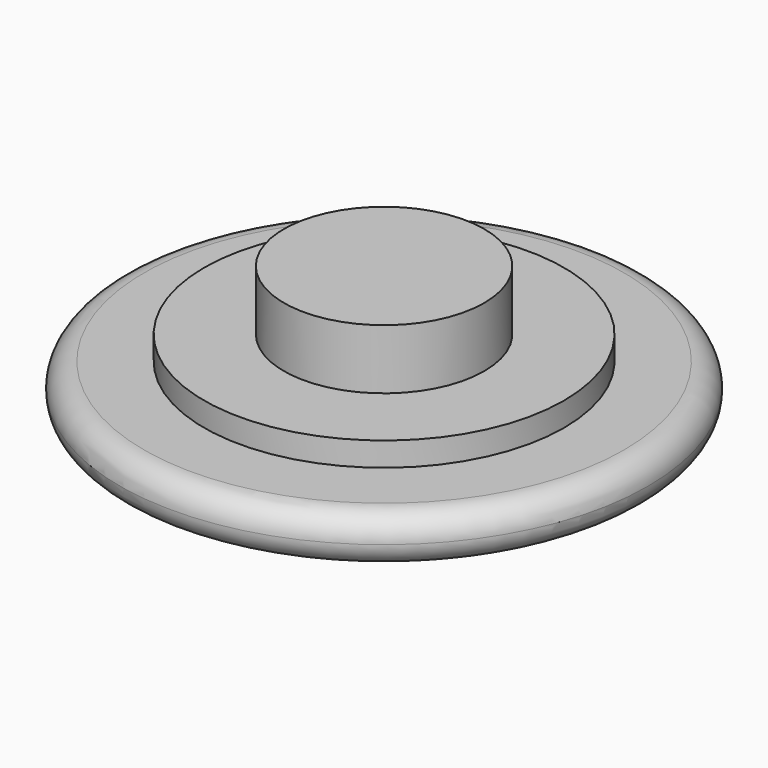
from build123d import *

# Parameters (mm, degrees)
F0_R         = 11
F0_R_2       = 7.5
F1_DEPTH     = 2
F0_R_3       = 4.175
F2_DEPTH     = 3
F3_DEPTH     = 5.5
F4_R         = 0.99999
F5_TEXT_SIZE = 5.9708603713
F6_DEPTH     = 1


# Not quite as in the source:
# - a fillet or chamfer is up to 0.001 mm smaller than in the source, because OpenCascade refuses the exact size
# - Text() gives the source's letters only with a copy of the font that has no kerning and outlines rounded to 1/6400 em; it was checked with that copy


with BuildPart() as f1:
    # F0 (on Top) → F1 (new body)
    with BuildSketch(Plane.XY):
        Circle(F0_R)
        Circle(F0_R_2, mode=Mode.SUBTRACT)
    extrude(amount=F1_DEPTH)

    # F0 (on Top) → F2 (join)
    with BuildSketch(Plane.XY):
        Circle(F0_R_2)
        Circle(F0_R_3, mode=Mode.SUBTRACT)
    extrude(amount=F2_DEPTH)

    # F0 (on Top) → F3 (join)
    with BuildSketch(Plane.XY):
        Circle(F0_R_3)
    extrude(amount=F3_DEPTH)

    # F4 (radius 1 in the source; OpenCascade refuses exactly that, so slightly less here)
    f4_edges = [f1.edges().sort_by_distance(p)[0] for p in [
        (-11, 0, 2),
        (-11, 0, 0),
    ]]
    fillet(f4_edges, radius=F4_R)

    # F5 (on face) → F6 (cut)
    with BuildSketch(Plane(origin=(0, 0, 0), x_dir=(1, 0, 0), z_dir=(0, 0, -1))):
        with Locations((-9.821636909, -1.8802788164)):
            Text('Paisley', F5_TEXT_SIZE, font='Open Sans', text_align=(TextAlign.LEFT, TextAlign.BOTTOM))
    extrude(amount=-F6_DEPTH, mode=Mode.SUBTRACT)


solid = f1.part
